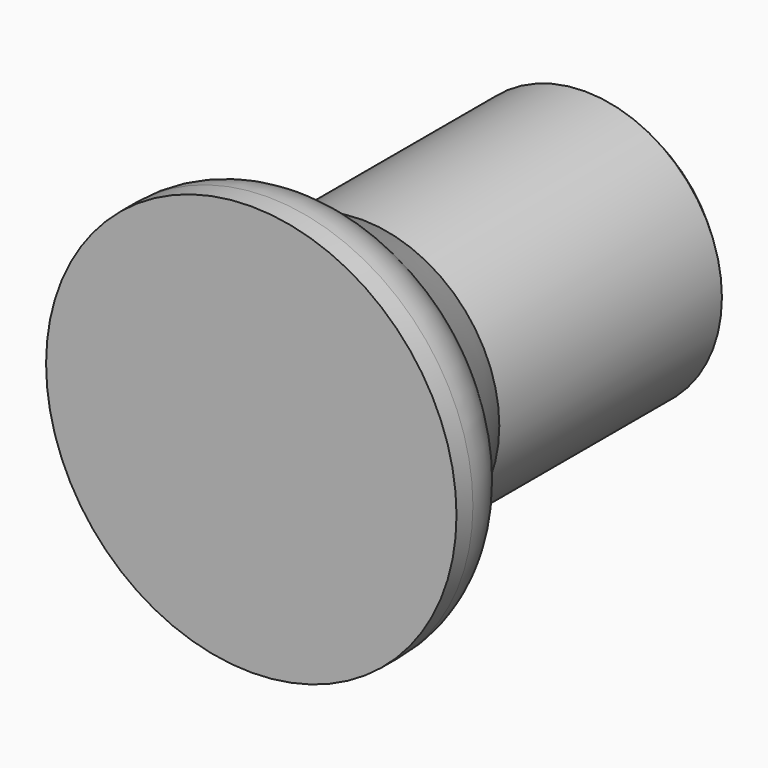
from build123d import *

# Parameters (mm, degrees)
F0_R        = 15
F1_DEPTH    = 6.5
F2_R        = 5
F3_R        = 10
F3_R_2      = 7.5
F4_DEPTH    = 25
F5_SIZE     = 1
F6_SIZE     = 1
F7_T2_ANGLE = 180
F7_T4_ANGLE = 180


# Not quite as in the source:
# - a fillet or chamfer that OpenCascade refuses, or shapes differently, is made with other operations: its cross-section is extruded or revolved along the edge and cut away or added


with BuildPart() as f1:
    # F0 (on Front) → F1 (new body)
    with BuildSketch(Plane.XZ):
        Circle(F0_R)
    extrude(amount=-F1_DEPTH)

    # F2
    f2_edges = [f1.edges().sort_by_distance(p)[0] for p in [
        (-15, 6.5, 0),
    ]]
    fillet(f2_edges, radius=F2_R)

    # F3 (on face) → F4 (join)
    with BuildSketch(Plane(origin=(0, 6.5, 0), x_dir=(-1, 0, 0), z_dir=(0, 1, 0))):
        Circle(F3_R)
        Circle(F3_R_2, mode=Mode.SUBTRACT)
    extrude(amount=F4_DEPTH)

    # F5
    f5_edges = [f1.edges().sort_by_distance(p)[0] for p in [
        (7.5, 31.5, 0),
    ]]
    chamfer(f5_edges, length=F5_SIZE)

    # F6
    f6_edges = [f1.edges().sort_by_distance(p)[0] for p in [
        (10, 31.5, 0),
    ]]
    chamfer(f6_edges, length=F6_SIZE)

    # F7: chamfer of 5 on 2 edges, made by hand

    # F7_s1 → F7_t2 (revolve)
    with BuildSketch(Plane.XY):
        with BuildLine():
            Line((10, 10.1602540378), (12.5, 5.8301270189))
            ThreePointArc((12.5, 5.8301270189), (11.3657058128, 6.3098698146), (10, 6.5))
            Line((10, 6.5), (10, 10.1602540378))
        make_face()
    revolve(axis=Axis((0, 6.5, 0), (0, -1, 0)), revolution_arc=F7_T2_ANGLE)

    # F7_s3 → F7_t4 (revolve)
    with BuildSketch(Plane.XY):
        with BuildLine():
            Line((-10, 10.1602540378), (-12.5, 5.8301270189))
            ThreePointArc((-12.5, 5.8301270189), (-11.3657058128, 6.3098698146), (-10, 6.5))
            Line((-10, 6.5), (-10, 10.1602540378))
        make_face()
    revolve(axis=Axis((0, 6.5, 0), (0, -1, 0)), revolution_arc=F7_T4_ANGLE)


solid = f1.part
